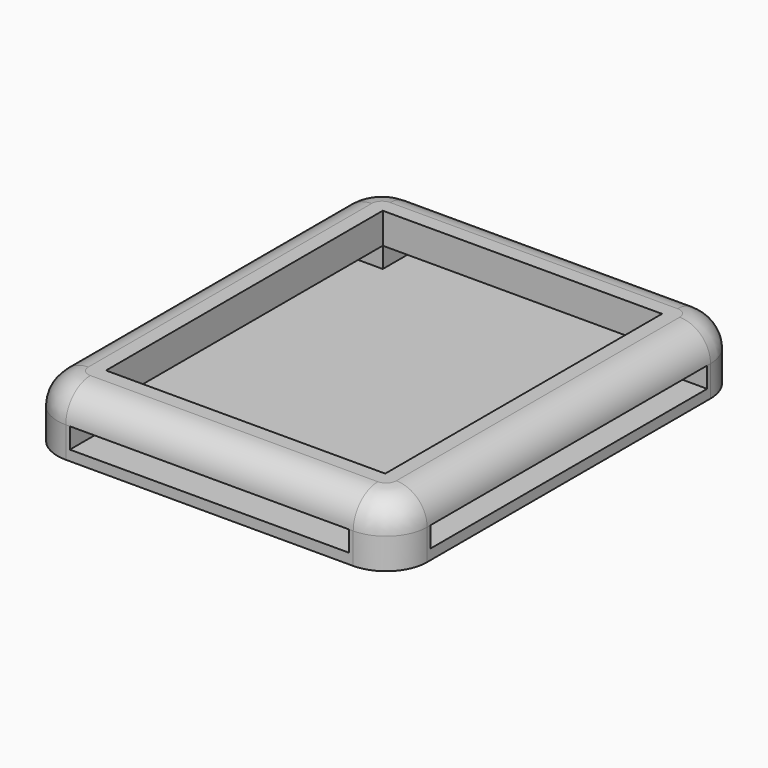
from build123d import *

# Parameters (mm, degrees)
F0_W         = 27.2
F0_H         = 4.4
F0_W_2       = 4.4
F0_H_2       = 33.7
F1_DEPTH     = 3
F2_R         = 2.99999
F3_DEPTH     = 2
F4_W         = 4.4
F4_H         = 4.4
F5_DEPTH     = 1
F6_T1_DEPTH  = 16
F6_T4_ANGLE  = 90
F6_T6_ANGLE  = 90
F6_T8_ANGLE  = 90
F6_T10_ANGLE = 90


# Not quite as in the source:
# - a fillet or chamfer that OpenCascade refuses, or shapes differently, is made with other operations: its cross-section is extruded or revolved along the edge and cut away or added
# - a fillet or chamfer is up to 0.001 mm smaller than in the source, because OpenCascade refuses the exact size


with BuildPart() as f1:
    # F0 (on Top) → F1 (new body)
    with BuildSketch(Plane.XY):
        with Locations((0.1669520199, 19.5440534235)):
            Rectangle(F0_W, F0_H)
        with Locations((-15.6330479801, 0.4940534235)):
            Rectangle(F0_W_2, F0_H_2)
        with Locations((-15.6330479801, 19.5440534235)):
            Rectangle(F0_W_2, F0_H)
        with Locations((-15.6330479801, -18.5559465765)):
            Rectangle(F0_W_2, F0_H)
        with Locations((0.1669520199, -18.5559465765)):
            Rectangle(F0_W, F0_H)
        with Locations((15.9669520199, -18.5559465765)):
            Rectangle(F0_W_2, F0_H)
        with Locations((15.9669520199, 0.4940534235)):
            Rectangle(F0_W_2, F0_H_2)
        with Locations((15.9669520199, 19.5440534235)):
            Rectangle(F0_W_2, F0_H)
    extrude(amount=F1_DEPTH)

    # F2 (radius 3 in the source; OpenCascade refuses exactly that, so slightly less here)
    f2_edges = [f1.edges().sort_by_distance(p)[0] for p in [
        (18.166952, 0.494053, 3),
        (0.166952, 21.744053, 3),
        (-17.833048, 0.494053, 3),
        (0.166952, -20.755947, 3),
    ]]
    fillet(f2_edges, radius=F2_R)

    # F0 (on Top) → F3 (join)
    with BuildSketch(Plane.XY):
        with Locations((-15.6330479801, -18.5559465765)):
            Rectangle(F0_W_2, F0_H)
        with Locations((15.9669520199, -18.5559465765)):
            Rectangle(F0_W_2, F0_H)
        with Locations((15.9669520199, 19.5440534235)):
            Rectangle(F0_W_2, F0_H)
        with Locations((-15.6330479801, 19.5440534235)):
            Rectangle(F0_W_2, F0_H)
    extrude(amount=-F3_DEPTH)

    # F4 (on face) → F5 (join)
    with BuildSketch(Plane(origin=(0, 0, -2), x_dir=(1, 0, 0), z_dir=(0, 0, -1))):
        Polygon((-13.4330479801, -21.7440534235), (18.1669520199, -21.7440534235), (18.1669520199, 20.7559465765), (-17.8330479801, 20.7559465765), (-17.8330479801, -17.3440534235), (-13.4330479801, -17.3440534235), align=None)
        with Locations((-15.6330479801, -19.5440534235)):
            Rectangle(F4_W, F4_H)
    extrude(amount=F5_DEPTH)

    # F6: fillet of radius 4 on 4 edges, made by hand

    # F6_s2 → F6_t1 (cut)
    with BuildSketch(Plane.XY.offset(-13)):
        with BuildLine():
            ThreePointArc((18.1669520199, 17.7440534235), (16.9953791447, 20.5724805482), (14.1669520199, 21.7440534235))
            Line((14.1669520199, 21.7440534235), (18.1669520199, 21.7440534235))
            Line((18.1669520199, 21.7440534235), (18.1669520199, 17.7440534235))
        make_face()
        with BuildLine():
            ThreePointArc((18.1669520199, -16.7559465765), (16.9953791447, -19.5843737013), (14.1669520199, -20.7559465765))
            Line((14.1669520199, -20.7559465765), (18.1669520199, -20.7559465765))
            Line((18.1669520199, -20.7559465765), (18.1669520199, -16.7559465765))
        make_face()
        with BuildLine():
            ThreePointArc((-17.8330479801, -16.7559465765), (-16.6614751048, -19.5843737013), (-13.8330479801, -20.7559465765))
            Line((-13.8330479801, -20.7559465765), (-17.8330479801, -20.7559465765))
            Line((-17.8330479801, -20.7559465765), (-17.8330479801, -16.7559465765))
        make_face()
        with BuildLine():
            ThreePointArc((-17.8330479801, 17.7440534235), (-16.6614751048, 20.5724805482), (-13.8330479801, 21.7440534235))
            Line((-13.8330479801, 21.7440534235), (-17.8330479801, 21.7440534235))
            Line((-17.8330479801, 21.7440534235), (-17.8330479801, 17.7440534235))
        make_face()
    extrude(amount=F6_T1_DEPTH, mode=Mode.SUBTRACT)

    # F6_s3 → F6_t4 (revolve, cut)
    with BuildSketch(Plane.YZ.offset(-13.8330479801)):
        with BuildLine():
            ThreePointArc((18.7440634235, 3), (20.8653766959, 2.1213232725), (21.7440534235, 1e-05))
            Line((21.7440534235, 1e-05), (21.7440534235, 3))
            Line((21.7440534235, 3), (18.7440634235, 3))
        make_face()
    revolve(axis=Axis((-13.8330479801, 17.7440534235, 3), (0, 0, 1)), revolution_arc=F6_T4_ANGLE, mode=Mode.SUBTRACT)

    # F6_s5 → F6_t6 (revolve, cut)
    with BuildSketch(Plane.XZ.offset(16.7559465765)):
        with BuildLine():
            ThreePointArc((-14.8330579801, 3), (-16.9543712526, 2.1213232725), (-17.8330479801, 1e-05))
            Line((-17.8330479801, 1e-05), (-17.8330479801, 3))
            Line((-17.8330479801, 3), (-14.8330579801, 3))
        make_face()
    revolve(axis=Axis((-13.8330479801, -16.7559465765, 3), (0, 0, 1)), revolution_arc=F6_T6_ANGLE, mode=Mode.SUBTRACT)

    # F6_s7 → F6_t8 (revolve, cut)
    with BuildSketch(Plane.YZ.offset(14.1669520199)):
        with BuildLine():
            ThreePointArc((-17.7559565765, 3), (-19.877269849, 2.1213232725), (-20.7559465765, 1e-05))
            Line((-20.7559465765, 1e-05), (-20.7559465765, 3))
            Line((-20.7559465765, 3), (-17.7559565765, 3))
        make_face()
    revolve(axis=Axis((14.1669520199, -16.7559465765, 3), (0, 0, 1)), revolution_arc=F6_T8_ANGLE, mode=Mode.SUBTRACT)

    # F6_s9 → F6_t10 (revolve, cut)
    with BuildSketch(Plane.XZ.offset(-17.7440534235)):
        with BuildLine():
            ThreePointArc((15.1669620199, 3), (17.2882752924, 2.1213232725), (18.1669520199, 1e-05))
            Line((18.1669520199, 1e-05), (18.1669520199, 3))
            Line((18.1669520199, 3), (15.1669620199, 3))
        make_face()
    revolve(axis=Axis((14.1669520199, 17.7440534235, 3), (0, 0, 1)), revolution_arc=F6_T10_ANGLE, mode=Mode.SUBTRACT)


solid = f1.part
